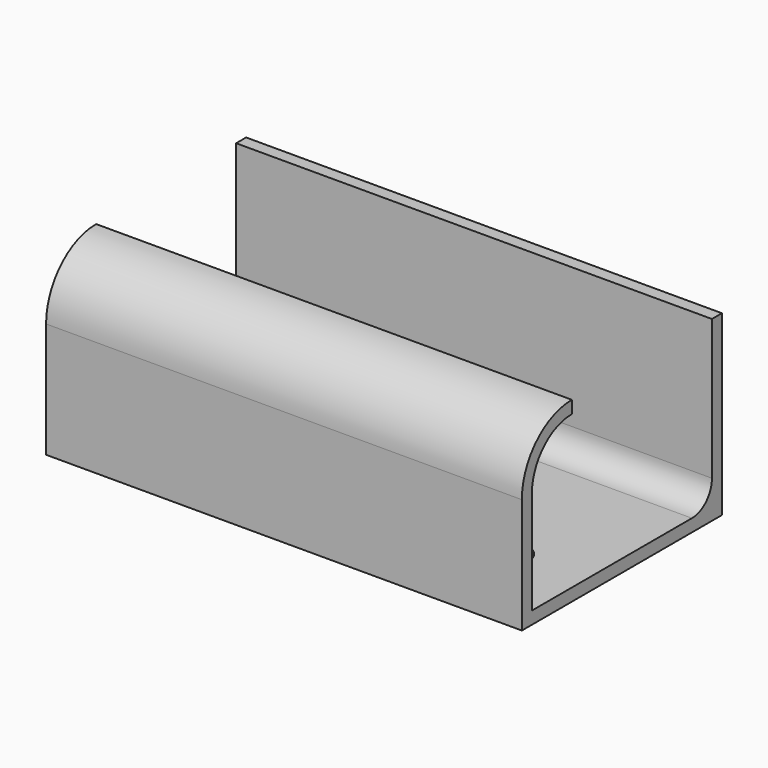
from build123d import *

# Parameters (mm, degrees)
F0_W     = 95.1395854354
F0_H     = 35.537417978
F1_DEPTH = 50
F2_R     = 12.5
F3_T     = 2.5
F4_R     = 5
F5_R     = 4.25
F6_DEPTH = 25


# Not quite as in the source:
# - a shell that OpenCascade refuses in one call is made with other operations: the cavity is built on its own and cut out


with BuildPart() as f1:
    # F0 (on Front) → F1 (new body)
    with BuildSketch(Plane.XZ):
        with Locations((-14.7300325334, 39.2820779234)):
            Rectangle(F0_W, F0_H)
    extrude(amount=-F1_DEPTH)

    # F2
    f2_edges = [f1.edges().sort_by_distance(p)[0] for p in [
        (-14.730033, 0, 57.050787),
    ]]
    fillet(f2_edges, radius=F2_R)

    # F3: shell of thickness 2.5, made by hand


with BuildPart() as f3_core1:
    # F3_t2: copy of F1
    add(f1.part)

    # the walls: a layer under each face that stays
    f3_faces = [f3_core1.faces().sort_by_distance(p)[0] for p in [
        (-14.7300325334, 3.6611652352, 53.3896216773),
        (-14.7300325334, 50, 39.2820779234),
        (-14.7300325334, 0, 33.0320779234),
        (-14.7300325334, 25, 21.5133689344),
    ]]
    thicken(f3_faces, amount=-F3_T, mode=Mode.SUBTRACT)


with BuildPart() as f1_1:
    add(f1.part)

    # what is left inside the walls is the cavity
    f3_cavity = [f3_core1.part.solids().sort_by_distance(p)[0] for p in [
        (-14.730033, 32.5, 24.038369),
    ]]
    add(f3_cavity, mode=Mode.SUBTRACT)

    # F4
    f4_edges = [f1_1.edges().sort_by_distance(p)[0] for p in [
        (-14.730033, 47.5, 24.013369),
    ]]
    fillet(f4_edges, radius=F4_R)

    # F5 (on face) → F6 (cut)
    with BuildSketch(Plane(origin=(0, 0, 21.5133689344), x_dir=(1, 0, 0), z_dir=(0, 0, -1))):
        with Locations((17.8397601843, -15)):
            Circle(F5_R)
    extrude(amount=-F6_DEPTH, mode=Mode.SUBTRACT)


solid = f1_1.part
